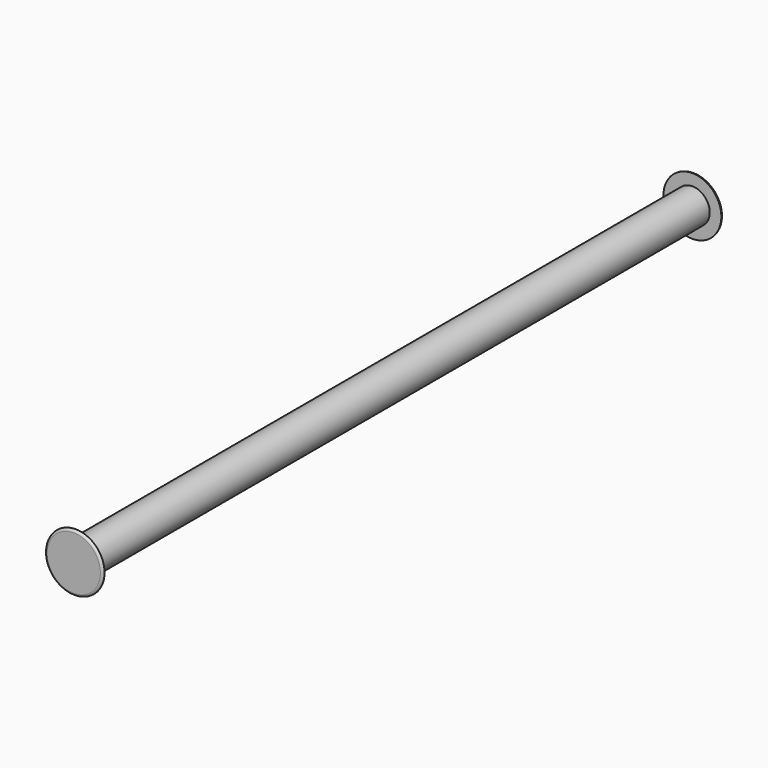
from build123d import *

# Parameters (mm, degrees)
F0_R     = 0.1905
F1_DEPTH = 8.4582
F2_R     = 0.3175
F3_DEPTH = 0.0254
F4_R     = 0.3175
F5_DEPTH = 0.0254
F6_R     = 0.02539
F7_R     = 0.02539


# Not quite as in the source:
# - a fillet or chamfer is up to 0.001 mm smaller than in the source, because OpenCascade refuses the exact size


with BuildPart() as f1:
    # F0 (on Front) → F1 (new body)
    with BuildSketch(Plane.XZ):
        Circle(F0_R)
    extrude(amount=F1_DEPTH)

    # F2 (on face) → F3 (join)
    with BuildSketch(Plane.XZ.offset(8.4582)):
        Circle(F2_R)
    extrude(amount=F3_DEPTH)

    # F4 (on face) → F5 (join)
    with BuildSketch(Plane(origin=(0, 0, 0), x_dir=(-1, 0, 0), z_dir=(0, 1, 0))):
        Circle(F4_R)
    extrude(amount=F5_DEPTH)

    # F6 (radius 0.0254 in the source; OpenCascade refuses exactly that, so slightly less here)
    f6_edges = [f1.edges().sort_by_distance(p)[0] for p in [
        (0.3175, 0.0254, 0),
    ]]
    fillet(f6_edges, radius=F6_R)

    # F7 (radius 0.0254 in the source; OpenCascade refuses exactly that, so slightly less here)
    f7_edges = [f1.edges().sort_by_distance(p)[0] for p in [
        (-0.3175, -8.4836, 0),
    ]]
    fillet(f7_edges, radius=F7_R)


solid = f1.part
